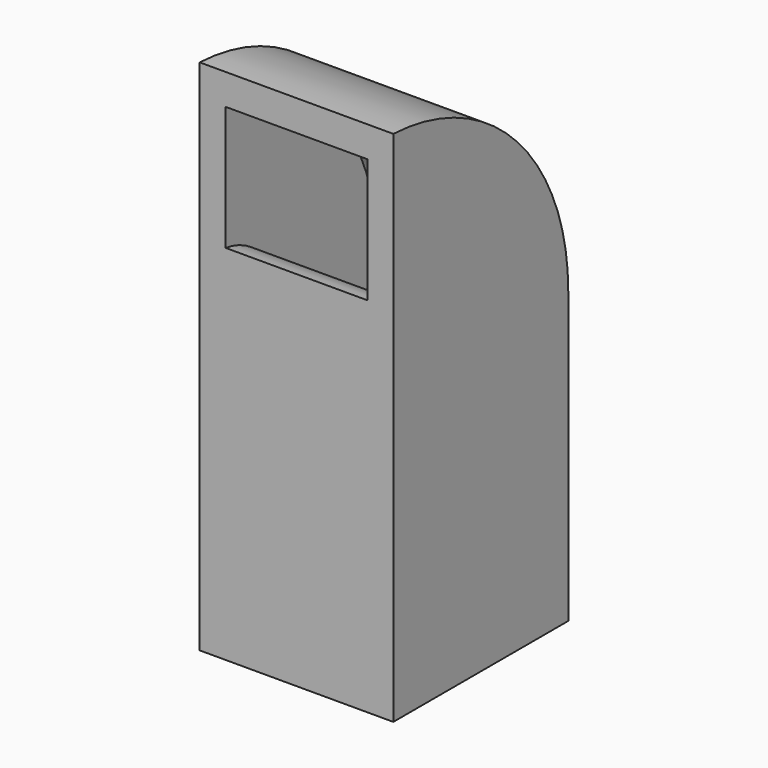
from build123d import *

# Parameters (mm, degrees)
F0_W        = 95.0020104647
F0_H        = 107.3112413287
F1_DEPTH    = 254
F2_T1_DEPTH = 655.5528673222
F3_W        = 69.5454850793
F3_H        = 60.9275996685


# Not quite as in the source:
# - a fillet or chamfer that OpenCascade refuses, or shapes differently, is made with other operations: its cross-section is extruded or revolved along the edge and cut away or added


with BuildPart() as f1:
    # F0 (on Top) → F1 (new body)
    with BuildSketch(Plane.XY):
        Rectangle(F0_W, F0_H)
    extrude(amount=F1_DEPTH)

    # F2: fillet of radius 112.2174748062 on 1 edges, made by hand

    # F2_s2 → F2_t1 (cut)
    with BuildSketch(Plane.YZ.offset(-327.7764336611)):
        with BuildLine():
            ThreePointArc((53.6556206644, 141.8898286285), (22.5039425406, 219.4855647234), (-53.6556206644, 254))
            Line((-53.6556206644, 254), (53.6556206644, 254))
            Line((53.6556206644, 254), (53.6556206644, 141.8898286285))
        make_face()
    extrude(amount=F2_T1_DEPTH, mode=Mode.SUBTRACT)

    # F4: sweep along a path in F4_path
    with BuildLine(Plane(origin=(-47.5010052323, -53.6556206644, 254), x_dir=(0, 0, 1), z_dir=(1, 0, 0))) as f4_path:
        ThreePointArc((0, 0), (-34.5144352766, -76.159563205), (-112.1101713715, -107.3112413288))
        Line((-112.1101713715, -107.3112413288), (-254, -107.3112413288))
    # F3 (on face) → F4 (sweep, cut)
    with BuildSketch(Plane.XZ.offset(53.6556206644)):
        with Locations((0, 208.4547877312)):
            Rectangle(F3_W, F3_H)
    sweep(path=f4_path.line, mode=Mode.SUBTRACT)


solid = f1.part
